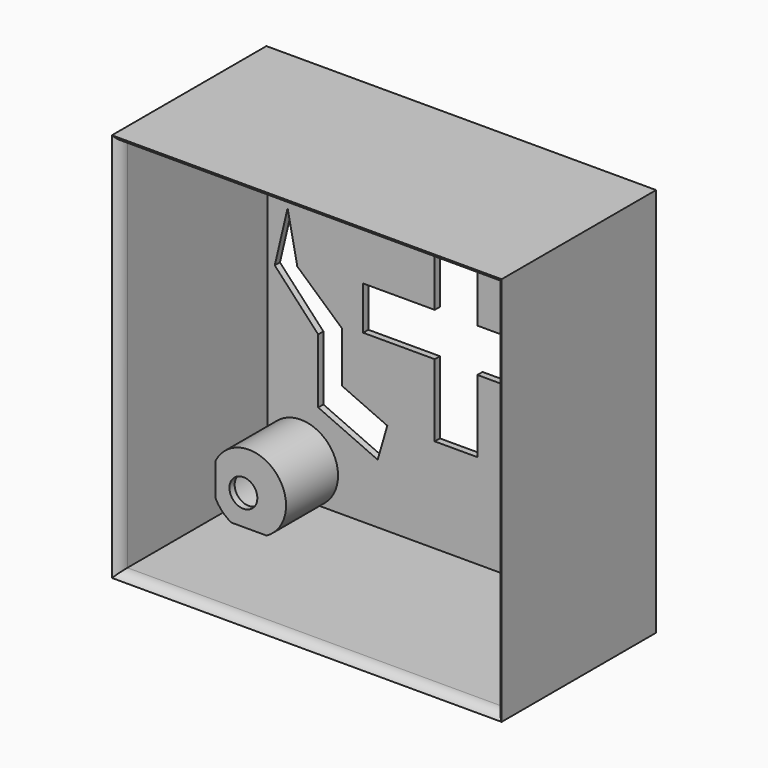
from build123d import *

# Parameters (mm, degrees)
F0_W         = 152.4
F0_H         = 152.4
F1_DEPTH     = 76.2
F2_R         = 12.8651099241
F2_R_2       = 12.0389782125
F2_R_3       = 13.4461105648
F2_R_4       = 11.9959461494
F3_DEPTH     = 25.4
F4_T         = 2.54
F5_T1_DEPTH  = 147.32
F5_T3_DEPTH  = 147.32
F5_T9_DEPTH  = 160.02
F5_T15_DEPTH = 160.02
F5_T24_DEPTH = 160.02
F5_T30_DEPTH = 160.02
F5_T39_DEPTH = 160.02
F5_T45_DEPTH = 160.02
F5_T54_DEPTH = 160.02
F5_T60_DEPTH = 160.02
F6_W         = 16.6622009128
F6_H         = 28.2943053171
F6_H_2       = 16.9765818864
F6_W_2       = 27.9799224809
F7_DEPTH     = 25.4
F8_R         = 5.4524649891
F8_R_2       = 5.9328095345
F8_R_3       = 6.7719768786
F8_R_4       = 7.5712998573
F9_DEPTH     = 25.4
F11_DEPTH    = 25.4


# Not quite as in the source:
# - a fillet or chamfer that OpenCascade refuses, or shapes differently, is made with other operations: its cross-section is extruded or revolved along the edge and cut away or added
# - a shell that OpenCascade refuses in one call is made with other operations: the cavity is built on its own and cut out


with BuildPart() as f1:
    # F0 (on Front) → F1 (new body)
    with BuildSketch(Plane.XZ):
        Rectangle(F0_W, F0_H)
    extrude(amount=F1_DEPTH)

    # F2 (on face) → F3 (cut)
    with BuildSketch(Plane.XZ):
        with Locations((57.6343238354, 59.4989620149)):
            Circle(F2_R)
        with Locations((-57.2953000665, 60.177013278)):
            Circle(F2_R_2)
        with Locations((58.6513988674, -59.8379895091)):
            Circle(F2_R_3)
        with Locations((-60.6855526567, -60.8550645411)):
            Circle(F2_R_4)
    extrude(amount=F3_DEPTH, mode=Mode.SUBTRACT)

    # F4: shell of thickness 2.54, made by hand


with BuildPart() as f4_core1:
    # F4_t2: copy of F1
    add(f1.part)

    # the walls: a layer under each face that stays
    f4_faces = [f4_core1.faces().sort_by_distance(p)[0] for p in [
        (0, -38.1, 76.2),
        (76.2, -38.1, 0),
        (-76.2, -38.1, 0),
        (0, 0, 0),
        (0, -38.1, -76.2),
        (-72.681498806, -12.7, -60.8550645411),
        (45.2052883026, -12.7, -59.8379895091),
        (-69.334278279, -12.7, 60.177013278),
        (44.7692139113, -12.7, 59.4989620149),
        (-60.6855526567, -25.4, -60.8550645411),
        (58.6513988674, -25.4, -59.8379895091),
        (-57.2953000665, -25.4, 60.177013278),
        (57.6343238354, -25.4, 59.4989620149),
    ]]
    thicken(f4_faces, amount=-F4_T, mode=Mode.SUBTRACT)

    # F4_s3 → F4_t4 (revolve, cut)
    with BuildSketch(Plane.XY.offset(-60.8550645411)):
        Polygon((-48.7150065073, -25.3746), (-46.1496065073, -25.4), (-46.1496065073, -27.94), (-48.6896065073, -27.94), align=None)
    revolve(axis=Axis((-60.6855526567, -25.4, -60.8550645411), (0, -1, 0)), mode=Mode.SUBTRACT)

    # F4_s5 → F4_t6 (revolve, cut)
    with BuildSketch(Plane.XY.offset(-59.8379895091)):
        Polygon((72.0721094321, -25.3746), (74.6375094321, -25.4), (74.6375094321, -27.94), (72.0975094321, -27.94), align=None)
    revolve(axis=Axis((58.6513988674, -25.4, -59.8379895091), (0, -1, 0)), mode=Mode.SUBTRACT)

    # F4_s7 → F4_t8 (revolve, cut)
    with BuildSketch(Plane.XY.offset(60.177013278)):
        Polygon((-45.281721854, -25.3746), (-42.716321854, -25.4), (-42.716321854, -27.94), (-45.256321854, -27.94), align=None)
    revolve(axis=Axis((-57.2953000665, -25.4, 60.177013278), (0, -1, 0)), mode=Mode.SUBTRACT)

    # F4_s9 → F4_t10 (revolve, cut)
    with BuildSketch(Plane.XY.offset(59.4989620149)):
        Polygon((70.4740337595, -25.3746), (73.0394337595, -25.4), (73.0394337595, -27.94), (70.4994337595, -27.94), align=None)
    revolve(axis=Axis((57.6343238354, -25.4, 59.4989620149), (0, -1, 0)), mode=Mode.SUBTRACT)


with BuildPart() as f1_1:
    add(f1.part)

    # what is left inside the walls is the cavity
    f4_cavity = [f4_core1.part.solids().sort_by_distance(p)[0] for p in [
        (0, -76.1746, -24.553333),
    ]]
    add(f4_cavity, mode=Mode.SUBTRACT)

    # F5: fillet of radius 5.08 on 4 edges, made by hand

    # F5_s2 → F5_t1 (cut)
    with BuildSketch(Plane.YZ.offset(-73.66)):
        with BuildLine():
            ThreePointArc((-76.2, 78.74), (-74.7121024484, 75.1478975516), (-71.12, 73.66))
            Line((-71.12, 73.66), (-76.2, 73.66))
            Line((-76.2, 73.66), (-76.2, 78.74))
        make_face()
        with BuildLine():
            ThreePointArc((-76.2, -78.74), (-74.7121024484, -75.1478975516), (-71.12, -73.66))
            Line((-71.12, -73.66), (-76.2, -73.66))
            Line((-76.2, -73.66), (-76.2, -78.74))
        make_face()
    extrude(amount=F5_T1_DEPTH, mode=Mode.SUBTRACT)

    # F5_s4 → F5_t3 (cut)
    with BuildSketch(Plane.XY.offset(-73.66)):
        with BuildLine():
            ThreePointArc((-78.74, -76.2), (-75.1478975516, -74.7121024484), (-73.66, -71.12))
            Line((-73.66, -71.12), (-73.66, -76.2))
            Line((-73.66, -76.2), (-78.74, -76.2))
        make_face()
        with BuildLine():
            ThreePointArc((78.74, -76.2), (75.1478975516, -74.7121024484), (73.66, -71.12))
            Line((73.66, -71.12), (73.66, -76.2))
            Line((73.66, -76.2), (78.74, -76.2))
        make_face()
    extrude(amount=F5_T3_DEPTH, mode=Mode.SUBTRACT)


with BuildPart() as f5_tool7:
    # F5_s8 → F5_t9 (new body)
    with BuildSketch(Plane.YZ.offset(86.36)):
        with BuildLine():
            ThreePointArc((-76.2, 78.74), (-74.7121024484, 75.1478975516), (-71.12, 73.66))
            Line((-71.12, 73.66), (-76.2, 73.66))
            Line((-76.2, 73.66), (-76.2, 78.74))
        make_face()
    extrude(amount=-F5_T9_DEPTH)

    split(bisect_by=Plane.XY.offset(76.2), keep=Keep.BOTTOM)

    split(bisect_by=Plane.YZ.offset(76.2), keep=Keep.BOTTOM)

    split(bisect_by=Plane.YZ.offset(73.66), keep=Keep.TOP)


with BuildPart() as f5_tool13:
    # F5_s14 → F5_t15 (new body)
    with BuildSketch(Plane.XY.offset(-73.66)):
        with BuildLine():
            ThreePointArc((78.74, -76.2), (75.1478975516, -74.7121024484), (73.66, -71.12))
            Line((73.66, -71.12), (73.66, -76.2))
            Line((73.66, -76.2), (78.74, -76.2))
        make_face()
    extrude(amount=F5_T15_DEPTH)

    split(bisect_by=Plane.XY.offset(76.2), keep=Keep.BOTTOM)

    split(bisect_by=Plane.YZ.offset(76.2), keep=Keep.BOTTOM)

    split(bisect_by=Plane.XY.offset(73.66), keep=Keep.TOP)


with BuildPart() as f5_tool7_1:
    add(f5_tool7.part)

    # F5_t19: intersect F5_tool13
    add(f5_tool13.part, mode=Mode.INTERSECT)


with BuildPart() as f1_2:
    add(f1_1.part)

    # F5_t5: cut F5_tool7
    add(f5_tool7_1.part, mode=Mode.SUBTRACT)


with BuildPart() as f5_tool22:
    # F5_s23 → F5_t24 (new body)
    with BuildSketch(Plane.YZ.offset(73.66)):
        with BuildLine():
            ThreePointArc((-76.2, 78.74), (-74.7121024484, 75.1478975516), (-71.12, 73.66))
            Line((-71.12, 73.66), (-76.2, 73.66))
            Line((-76.2, 73.66), (-76.2, 78.74))
        make_face()
    extrude(amount=-F5_T24_DEPTH)

    split(bisect_by=Plane.XY.offset(76.2), keep=Keep.BOTTOM)

    split(bisect_by=Plane.YZ.offset(-76.2), keep=Keep.TOP)

    split(bisect_by=Plane.YZ.offset(-73.66), keep=Keep.BOTTOM)


with BuildPart() as f5_tool28:
    # F5_s29 → F5_t30 (new body)
    with BuildSketch(Plane.XY.offset(86.36)):
        with BuildLine():
            ThreePointArc((-78.74, -76.2), (-75.1478975516, -74.7121024484), (-73.66, -71.12))
            Line((-73.66, -71.12), (-73.66, -76.2))
            Line((-73.66, -76.2), (-78.74, -76.2))
        make_face()
    extrude(amount=-F5_T30_DEPTH)

    split(bisect_by=Plane.XY.offset(76.2), keep=Keep.BOTTOM)

    split(bisect_by=Plane.YZ.offset(-76.2), keep=Keep.TOP)

    split(bisect_by=Plane.XY.offset(73.66), keep=Keep.TOP)


with BuildPart() as f5_tool22_1:
    add(f5_tool22.part)

    # F5_t34: intersect F5_tool28
    add(f5_tool28.part, mode=Mode.INTERSECT)


with BuildPart() as f1_3:
    add(f1_2.part)

    # F5_t20: cut F5_tool22
    add(f5_tool22_1.part, mode=Mode.SUBTRACT)


with BuildPart() as f5_tool37:
    # F5_s38 → F5_t39 (new body)
    with BuildSketch(Plane.XY.offset(73.66)):
        with BuildLine():
            ThreePointArc((-78.74, -76.2), (-75.1478975516, -74.7121024484), (-73.66, -71.12))
            Line((-73.66, -71.12), (-73.66, -76.2))
            Line((-73.66, -76.2), (-78.74, -76.2))
        make_face()
    extrude(amount=-F5_T39_DEPTH)

    split(bisect_by=Plane.YZ.offset(-76.2), keep=Keep.TOP)

    split(bisect_by=Plane.XY.offset(-76.2), keep=Keep.TOP)

    split(bisect_by=Plane.XY.offset(-73.66), keep=Keep.BOTTOM)


with BuildPart() as f5_tool43:
    # F5_s44 → F5_t45 (new body)
    with BuildSketch(Plane.YZ.offset(-86.36)):
        with BuildLine():
            ThreePointArc((-76.2, -78.74), (-74.7121024484, -75.1478975516), (-71.12, -73.66))
            Line((-71.12, -73.66), (-76.2, -73.66))
            Line((-76.2, -73.66), (-76.2, -78.74))
        make_face()
    extrude(amount=F5_T45_DEPTH)

    split(bisect_by=Plane.YZ.offset(-76.2), keep=Keep.TOP)

    split(bisect_by=Plane.XY.offset(-76.2), keep=Keep.TOP)

    split(bisect_by=Plane.YZ.offset(-73.66), keep=Keep.BOTTOM)


with BuildPart() as f5_tool37_1:
    add(f5_tool37.part)

    # F5_t49: intersect F5_tool43
    add(f5_tool43.part, mode=Mode.INTERSECT)


with BuildPart() as f1_4:
    add(f1_3.part)

    # F5_t35: cut F5_tool37
    add(f5_tool37_1.part, mode=Mode.SUBTRACT)


with BuildPart() as f5_tool52:
    # F5_s53 → F5_t54 (new body)
    with BuildSketch(Plane.YZ.offset(-73.66)):
        with BuildLine():
            ThreePointArc((-76.2, -78.74), (-74.7121024484, -75.1478975516), (-71.12, -73.66))
            Line((-71.12, -73.66), (-76.2, -73.66))
            Line((-76.2, -73.66), (-76.2, -78.74))
        make_face()
    extrude(amount=F5_T54_DEPTH)

    split(bisect_by=Plane.YZ.offset(76.2), keep=Keep.BOTTOM)

    split(bisect_by=Plane.XY.offset(-76.2), keep=Keep.TOP)

    split(bisect_by=Plane.YZ.offset(73.66), keep=Keep.TOP)


with BuildPart() as f5_tool58:
    # F5_s59 → F5_t60 (new body)
    with BuildSketch(Plane.XY.offset(-86.36)):
        with BuildLine():
            ThreePointArc((78.74, -76.2), (75.1478975516, -74.7121024484), (73.66, -71.12))
            Line((73.66, -71.12), (73.66, -76.2))
            Line((73.66, -76.2), (78.74, -76.2))
        make_face()
    extrude(amount=F5_T60_DEPTH)

    split(bisect_by=Plane.YZ.offset(76.2), keep=Keep.BOTTOM)

    split(bisect_by=Plane.XY.offset(-76.2), keep=Keep.TOP)

    split(bisect_by=Plane.XY.offset(-73.66), keep=Keep.BOTTOM)


with BuildPart() as f5_tool52_1:
    add(f5_tool52.part)

    # F5_t64: intersect F5_tool58
    add(f5_tool58.part, mode=Mode.INTERSECT)


with BuildPart() as f1_5:
    add(f1_4.part)

    # F5_t50: cut F5_tool52
    add(f5_tool52_1.part, mode=Mode.SUBTRACT)

    # F6 (on face) → F7 (cut)
    with BuildSketch(Plane.XZ.offset(2.54)):
        with Locations((0, 22.6354436018)):
            Rectangle(F6_W, F6_H)
        Rectangle(F6_W, F6_H_2)
        with Locations((0, -22.6354436018)):
            Rectangle(F6_W, F6_H)
        with Locations((22.3210616969, 0)):
            Rectangle(F6_W_2, F6_H_2)
        with Locations((-22.3210616969, 0)):
            Rectangle(F6_W_2, F6_H_2)
    extrude(amount=-F7_DEPTH, mode=Mode.SUBTRACT)

    # F8 (on face) → F9 (cut)
    with BuildSketch(Plane.XZ.offset(27.94)):
        with Locations((-62.8410799733, -61.9330853224)):
            Circle(F8_R)
        with Locations((-57.2953000665, 60.177013278)):
            Circle(F8_R_2)
        with Locations((56.4314164221, 60.6755614281)):
            Circle(F8_R_3)
        with Locations((58.3177022636, -59.4180375338)):
            Circle(F8_R_4)
    extrude(amount=-F9_DEPTH, mode=Mode.SUBTRACT)

    # F10 (on face) → F11 (cut)
    with BuildSketch(Plane.XZ):
        Polygon((17.9349766593, -45.055488267), (30.337780714, -50.615362823), (38.728027374, -30.3751360907), (52.3444600403, 0), (31.5953046083, 21.0635364056), (41.6555032134, 3.458192572), (36.6254039109, -21.6922983527), align=None)
        Polygon((-30.652159825, -50.3551833958), (-26.879588142, -37.4113582075), (-44.5359825398, -29.4964272347), (-44.5359825398, -9.7458148375), (-62.0902739465, 5.9732417576), (-65.8628493547, 24.8361118138), (-70.892944932, 3.458192572), (-53.9163686335, -14.7759132087), (-53.9163686335, -39.9264059961), align=None)
        Polygon((-42.5986461341, 40.5551679432), (-30.652159825, 35.5250686407), (-24.3645366281, 49.3578389287), (-24.3645366281, 59.4180375338), (-13.6755788699, 71.3645219803), (-31.9096893072, 63.8193711638), (-31.9096893072, 51.8728867173), align=None)
        Polygon((32.2240665555, 31.7524932325), (38.9561592304, 39.308484465), (34.110352397, 50.615362823), (20.2775839716, 50.615362823), (13.3611978963, 63.1906092167), (0, 66.334426403), (7.7023385093, 53.1304106116), (25.9364452213, 44.9565052986), align=None)
    extrude(amount=F11_DEPTH, mode=Mode.SUBTRACT)


solid = f1_5.part
